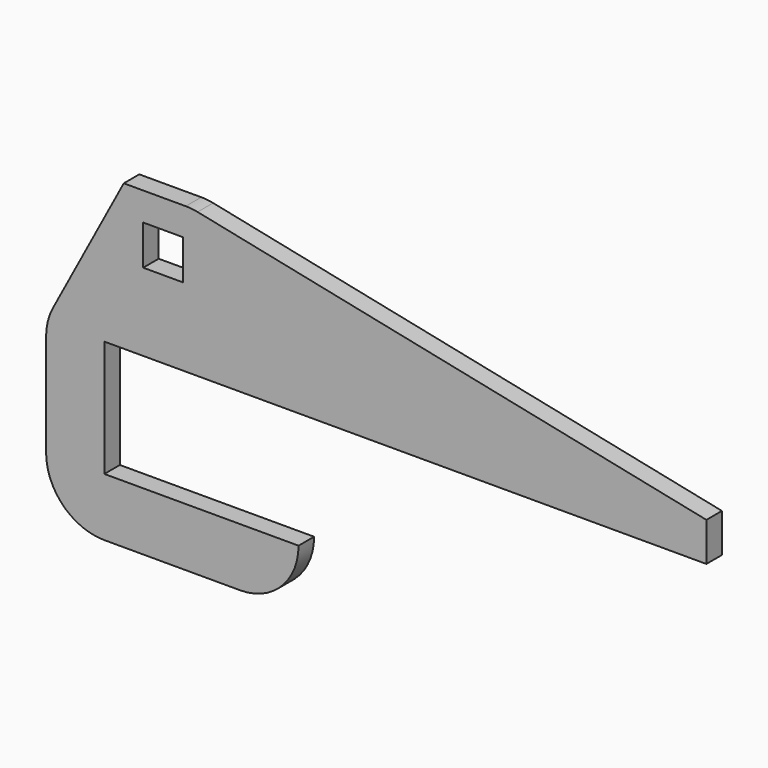
from build123d import *

# Parameters (mm, degrees)
F1_DEPTH = 6.35
F2_W     = 13.0048
F2_H     = 13.0048
F3_DEPTH = 6.351
F4_R     = 19.04999


# Not quite as in the source:
# - a fillet or chamfer is up to 0.001 mm smaller than in the source, because OpenCascade refuses the exact size


with BuildPart() as f1:
    # F0 (on Front) → F1 (new body)
    with BuildSketch(Plane.XZ):
        Polygon((0, 57.15), (0, 0), (82.55, 0), (82.55, 19.05), (19.05, 19.05), (19.05, 57.15), (215.9, 57.15), (215.9, 69.85), (47.625, 104.775), (25.4, 104.775), align=None)
    extrude(amount=F1_DEPTH)

    # F2 (on face) → F3 (cut, through all)
    with BuildSketch(Plane.XZ.offset(6.35)):
        with Locations((38.2524, 89.0524)):
            Rectangle(F2_W, F2_H)
    extrude(amount=-F3_DEPTH, mode=Mode.SUBTRACT)

    # F4 (radius 19.05 in the source; OpenCascade refuses exactly that, so slightly less here)
    f4_edges = [f1.edges().sort_by_distance(p)[0] for p in [
        (0, -3.175, 0),
        (82.55, -3.175, 0),
        (0, -3.175, 57.15),
        (47.625, -3.175, 104.775),
    ]]
    fillet(f4_edges, radius=F4_R)


solid = f1.part
